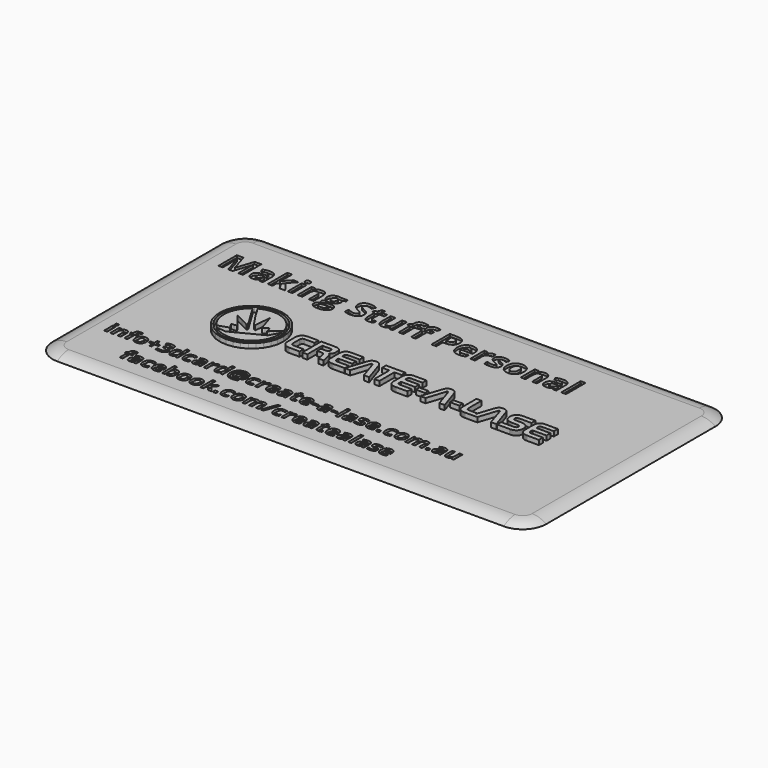
from build123d import *

# Parameters (mm, degrees)
F1_DEPTH     = 1
F0_W         = 1.9434
F0_H         = 0.9282
F4_DEPTH     = 1
F3_TEXT_SIZE = 4.3575753724
F5_DEPTH     = 0.5
F6_TEXT_SIZE = 6.8351726593
F7_DEPTH     = 0.5
F8_T1_DEPTH  = 45
F8_T3_DEPTH  = 95
F8_T6_ANGLE  = 90
F8_T8_ANGLE  = 90
F8_T10_ANGLE = 90
F8_T12_ANGLE = 90


# Not quite as in the source:
# - a fillet or chamfer that OpenCascade refuses, or shapes differently, is made with other operations: its cross-section is extruded or revolved along the edge and cut away or added
# - Text() gives the source's letters only with a copy of the font that has no kerning and outlines rounded to 1/6400 em; it was checked with that copy


with BuildPart() as f1:
    # F0 (on Top) → F1 (new body)
    with BuildSketch(Plane.XY):
        Polygon((-26.8391, 6.60025), (-28.2079, 6.73715), (-29.5767, 6.60025), (-30.8517, 6.20765), (-32.0054, 5.58655), (-33.0107, 4.76385), (-33.8401, 3.76675), (-34.4663, 2.62235), (-34.8621, 1.35775), (-35.0001, 5e-05), (-34.8621, -1.35765), (-34.4663, -2.62235), (-33.8401, -3.76675), (-33.0107, -4.76385), (-32.0054, -5.58655), (-30.8517, -6.20765), (-29.5767, -6.60025), (-28.2079, -6.73715), (-26.8391, -6.60025), (-25.5641, -6.20765), (-24.4103, -5.58655), (-23.4051, -4.76385), (-22.5757, -3.76675), (-21.9494, -2.62235), (-21.5536, -1.35765), (-21.4156, 5e-05), (-21.5536, 1.35775), (-21.9494, 2.62235), (-22.5757, 3.76675), (-23.4051, 4.76385), (-24.4103, 5.58655), (-25.5641, 6.20765), align=None)
        Polygon((-26.9199, -6.21065), (-28.2079, -6.33945), (-29.496, -6.21065), (-30.6957, -5.84125), (-31.7813, -5.25675), (-32.7272, -4.48265), (-33.5077, -3.54445), (-34.0969, -2.46755), (-34.4694, -1.27755), (-34.5992, 5e-05), (-34.4694, 1.27695), (-34.0969, 2.46635), (-33.5077, 3.54275), (-32.7272, 4.48075), (-31.7813, 5.25465), (-30.6957, 5.83905), (-29.496, 6.20845), (-28.2079, 6.33725), (-26.9199, 6.20845), (-25.7205, 5.83905), (-24.6352, 5.25465), (-23.6897, 4.48075), (-22.9096, 3.54275), (-22.3207, 2.46635), (-21.9486, 1.27695), (-21.8188, 5e-05), (-21.9486, -1.27755), (-22.3207, -2.46755), (-22.9096, -3.54445), (-23.6897, -4.48265), (-24.6352, -5.25675), (-25.7205, -5.84125), align=None, mode=Mode.SUBTRACT)
    extrude(amount=F1_DEPTH)



with BuildPart() as f1b:
    # F0 (on Top) → F1, piece 2 (new body)
    with BuildSketch(Plane.XY):
        Polygon((-15.8894, 2.46555), (-18.1095, 2.46555), (-18.2886, 2.45905), (-18.4578, 2.43955), (-18.617, 2.40695), (-18.7664, 2.36145), (-18.9057, 2.30295), (-19.0351, 2.23145), (-19.1544, 2.14705), (-19.2637, 2.04975), (-19.3618, 1.94045), (-19.4468, 1.82115), (-19.5187, 1.69165), (-19.5775, 1.55215), (-19.6231, 1.40255), (-19.6557, 1.24285), (-19.6753, 1.07305), (-19.6818, 0.89315), (-19.6818, -0.98735), (-19.6753, -1.16725), (-19.6557, -1.33725), (-19.6231, -1.49725), (-19.5775, -1.64725), (-19.5187, -1.78725), (-19.4468, -1.91735), (-19.3618, -2.03745), (-19.2637, -2.14755), (-19.1544, -2.24575), (-19.0351, -2.33085), (-18.9057, -2.40295), (-18.7664, -2.46195), (-18.617, -2.50785), (-18.4578, -2.54065), (-18.2886, -2.56035), (-18.1095, -2.56695), (-15.8894, -2.56695), (-15.8894, -1.50825), (-18.0068, -1.50825), (-18.1464, -1.49875), (-18.2678, -1.47015), (-18.3712, -1.42255), (-18.4564, -1.35595), (-18.523, -1.27075), (-18.5706, -1.16745), (-18.5991, -1.04595), (-18.6086, -0.90635), (-18.6086, 0.80495), (-18.5991, 0.94635), (-18.5706, 1.06945), (-18.523, 1.17425), (-18.4564, 1.26055), (-18.3712, 1.32795), (-18.2678, 1.37585), (-18.1464, 1.40455), (-18.0068, 1.41405), (-15.8894, 1.41405), align=None)
    extrude(amount=F1_DEPTH)


with BuildPart() as f1c:
    # F0 (on Top) → F1, piece 3 (new body)
    with BuildSketch(Plane.XY):
        Polygon((-12.5597, 2.46555), (-15.337, 2.46555), (-15.337, -2.56695), (-14.2638, -2.56695), (-14.2638, 1.41405), (-12.6057, 1.41405), (-12.4903, 1.40815), (-12.389, 1.39055), (-12.3018, 1.36105), (-12.2286, 1.31985), (-12.1706, 1.26775), (-12.1291, 1.20575), (-12.1041, 1.13405), (-12.0957, 1.05275), (-12.0957, 0.78195), (-12.1041, 0.70065), (-12.1291, 0.62895), (-12.1706, 0.56695), (-12.2286, 0.51485), (-12.3018, 0.47365), (-12.389, 0.44415), (-12.4903, 0.42655), (-12.6057, 0.42065), (-13.7562, 0.42065), (-13.7562, -0.58735), (-12.6758, -0.58735), (-12.5851, -0.59775), (-12.4999, -0.62925), (-12.4201, -0.68165), (-12.3458, -0.75535), (-12.2796, -0.84665), (-12.226, -0.95185), (-12.1849, -1.07085), (-12.1561, -1.20365), (-11.9083, -2.56695), (-10.7759, -2.56695), (-11.1397, -0.87015), (-11.3379, -0.38065), (-11.4113, -0.28985), (-11.4936, -0.21315), (-11.5848, -0.15065), (-11.6847, -0.10265), (-11.5272, -0.04125), (-11.3917, 0.03965), (-11.2779, 0.13995), (-11.1856, 0.25985), (-11.1142, 0.40125), (-11.0633, 0.56445), (-11.0327, 0.74935), (-11.0225, 0.95605), (-11.0225, 1.35725), (-11.0284, 1.49445), (-11.046, 1.62225), (-11.0754, 1.74075), (-11.1166, 1.84995), (-11.1694, 1.94995), (-11.234, 2.04065), (-11.3103, 2.12235), (-11.3983, 2.19485), (-11.4985, 2.25815), (-11.6116, 2.31305), (-11.7374, 2.35965), (-11.8761, 2.39775), (-12.1921, 2.44855), align=None)
    extrude(amount=F1_DEPTH)


with BuildPart() as f1d:
    # F0 (on Top) → F1, piece 4 (new body)
    with BuildSketch(Plane.XY):
        Polygon((-6.3018, 2.46555), (-8.7902, 2.46555), (-8.9959, 2.45995), (-9.1861, 2.44315), (-9.3609, 2.41505), (-9.5202, 2.37575), (-9.6641, 2.32535), (-9.7926, 2.26355), (-9.9058, 2.19065), (-10.0036, 2.10655), (-10.0877, 2.00875), (-10.1606, 1.89555), (-10.2223, 1.76705), (-10.2728, 1.62315), (-10.312, 1.46385), (-10.3401, 1.28905), (-10.3569, 1.09885), (-10.3625, 0.89315), (-10.3625, -0.98735), (-10.3568, -1.19315), (-10.3399, -1.38345), (-10.3116, -1.55855), (-10.272, -1.71825), (-10.2212, -1.86265), (-10.1591, -1.99175), (-10.0858, -2.10565), (-10.0012, -2.20435), (-9.9034, -2.28935), (-9.7902, -2.36295), (-9.6618, -2.42525), (-9.5181, -2.47625), (-9.359, -2.51595), (-9.1847, -2.54425), (-8.9951, -2.56125), (-8.7902, -2.56695), (-6.3018, -2.56695), (-6.3018, -1.50825), (-8.7092, -1.50825), (-8.8622, -1.50055), (-8.9892, -1.47725), (-9.0901, -1.43835), (-9.1649, -1.38375), (-9.2195, -1.30895), (-9.2583, -1.20795), (-9.2816, -1.08055), (-9.2893, -0.92695), (-9.2893, -0.55105), (-6.3018, -0.55105), (-6.3018, 0.50765), (-9.2893, 0.50765), (-9.2893, 0.82675), (-9.2814, 0.98145), (-9.2577, 1.11005), (-9.2184, 1.21245), (-9.1636, 1.28835), (-9.0882, 1.34315), (-8.9872, 1.38245), (-8.8608, 1.40615), (-8.7092, 1.41405), (-6.3018, 1.41405), align=None)
    extrude(amount=F1_DEPTH)


with BuildPart() as f1e:
    # F0 (on Top) → F1, piece 5 (new body)
    with BuildSketch(Plane.XY):
        Polygon((-1.0953, -2.56695), (-2.4875, 1.63885), (-2.565, 1.85635), (-2.6632, 2.04495), (-2.7821, 2.20445), (-2.9214, 2.33495), (-3.0816, 2.43645), (-3.2633, 2.50905), (-3.4664, 2.55255), (-3.6913, 2.56705), (-3.9154, 2.55325), (-4.1162, 2.51175), (-4.2938, 2.44265), (-4.4478, 2.34585), (-4.5826, 2.21875), (-4.7024, 2.05855), (-4.8069, 1.86525), (-4.8962, 1.63885), (-6.28, -2.56695), (-5.1403, -2.56695), (-3.8786, 1.33435), (-3.8061, 1.46725), (-3.6913, 1.50835), (-3.5692, 1.46605), (-3.493, 1.33185), (-2.2325, -2.56695), align=None)
    extrude(amount=F1_DEPTH)


with BuildPart() as f1f:
    # F0 (on Top) → F1, piece 6 (new body)
    with BuildSketch(Plane.XY):
        Polygon((2.5922, 2.46555), (-1.5339, 2.46555), (-1.5339, 1.41405), (-0.0038, 1.41405), (-0.0038, -2.56695), (1.0694, -2.56695), (1.0694, 1.41405), (2.5922, 1.41405), align=None)
    extrude(amount=F1_DEPTH)


with BuildPart() as f1g:
    # F0 (on Top) → F1, piece 7 (new body)
    with BuildSketch(Plane.XY):
        Polygon((7.0602, 2.46555), (4.5718, 2.46555), (4.3661, 2.45995), (4.1759, 2.44315), (4.0011, 2.41505), (3.8418, 2.37575), (3.6979, 2.32535), (3.5694, 2.26355), (3.4562, 2.19065), (3.3584, 2.10655), (3.2743, 2.00875), (3.2014, 1.89555), (3.1397, 1.76705), (3.0892, 1.62315), (3.05, 1.46385), (3.0219, 1.28905), (3.0051, 1.09885), (2.9995, 0.89315), (2.9995, -0.98735), (3.0052, -1.19315), (3.0221, -1.38345), (3.0504, -1.55855), (3.09, -1.71825), (3.1408, -1.86265), (3.2029, -1.99175), (3.2762, -2.10565), (3.3608, -2.20435), (3.4586, -2.28935), (3.5718, -2.36295), (3.7002, -2.42525), (3.8439, -2.47625), (4.003, -2.51595), (4.1773, -2.54425), (4.3669, -2.56125), (4.5718, -2.56695), (7.0602, -2.56695), (7.0602, -1.50825), (4.6528, -1.50825), (4.4998, -1.50055), (4.3728, -1.47725), (4.2719, -1.43835), (4.1971, -1.38375), (4.1425, -1.30895), (4.1037, -1.20795), (4.0804, -1.08055), (4.0727, -0.92695), (4.0727, -0.55105), (7.0602, -0.55105), (7.0602, 0.50765), (4.0727, 0.50765), (4.0727, 0.82675), (4.0806, 0.98145), (4.1043, 1.11005), (4.1436, 1.21245), (4.1984, 1.28835), (4.2738, 1.34315), (4.3748, 1.38245), (4.5012, 1.40615), (4.6528, 1.41405), (7.0602, 1.41405), align=None)
    extrude(amount=F1_DEPTH)


with BuildPart() as f1h:
    # F0 (on Top) → F1, piece 8 (new body)
    with BuildSketch(Plane.XY):
        with Locations((8.7063, -0.74685)):
            Rectangle(F0_W, F0_H)
    extrude(amount=F1_DEPTH)


with BuildPart() as f1i:
    # F0 (on Top) → F1, piece 9 (new body)
    with BuildSketch(Plane.XY):
        Polygon((14.9509, -2.56695), (13.5587, 1.63885), (13.4812, 1.85635), (13.383, 2.04495), (13.2641, 2.20445), (13.1248, 2.33495), (12.9646, 2.43645), (12.7829, 2.50905), (12.5798, 2.55255), (12.3549, 2.56705), (12.1308, 2.55325), (11.93, 2.51175), (11.7524, 2.44265), (11.5984, 2.34585), (11.4636, 2.21875), (11.3438, 2.05855), (11.2393, 1.86525), (11.15, 1.63885), (9.7662, -2.56695), (10.9059, -2.56695), (12.1676, 1.33435), (12.2401, 1.46725), (12.3549, 1.50835), (12.477, 1.46605), (12.5532, 1.33185), (13.8137, -2.56695), align=None)
    extrude(amount=F1_DEPTH)


with BuildPart() as f1j:
    # F0 (on Top) → F1, piece 10 (new body)
    with BuildSketch(Plane.XY):
        with Locations((16.0109, -0.74685)):
            Rectangle(F0_W, F0_H)
    extrude(amount=F1_DEPTH)


with BuildPart() as f1k:
    # F0 (on Top) → F1, piece 11 (new body)
    with BuildSketch(Plane.XY):
        Polygon((18.7604, 2.46555), (17.6872, 2.46555), (17.6872, -0.98735), (17.6929, -1.19315), (17.7101, -1.38345), (17.7386, -1.55855), (17.7786, -1.71825), (17.8299, -1.86265), (17.8927, -1.99175), (17.9667, -2.10565), (18.0522, -2.20435), (18.1509, -2.28935), (18.265, -2.36295), (18.3943, -2.42525), (18.5389, -2.47625), (18.6989, -2.51595), (18.8741, -2.54425), (19.0646, -2.56125), (19.2704, -2.56695), (20.7606, -2.56695), (20.9793, -1.902252457), (20.9793, -1.50825), (19.3477, -1.50825), (19.1946, -1.50035), (19.0668, -1.47665), (18.9643, -1.43735), (18.8873, -1.38255), (18.8318, -1.30715), (18.7921, -1.20595), (18.7683, -1.07915), (18.7604, -0.92695), align=None)
        Polygon((22.1444, 1.63885), (20.9793, -1.902252457), (20.9793, -2.56695), (21.9003, -2.56695), (23.162, 1.33435), (23.2345, 1.46725), (23.3493, 1.50835), (23.4714, 1.46605), (23.5476, 1.33185), (24.8082, -2.56695), (25.9454, -2.56695), (24.5531, 1.63885), (24.4756, 1.85635), (24.3774, 2.04495), (24.2585, 2.20445), (24.1192, 2.33495), (23.959, 2.43645), (23.7773, 2.50905), (23.5742, 2.55255), (23.3493, 2.56705), (23.1252, 2.55325), (22.9244, 2.51175), (22.7468, 2.44265), (22.5928, 2.34585), (22.458, 2.21875), (22.3382, 2.05855), (22.2337, 1.86525), align=None)
        Polygon((20.9793, -2.56695), (20.9793, -1.902252457), (20.7606, -2.56695), align=None)
    extrude(amount=F1_DEPTH)


with BuildPart() as f1l:
    # F0 (on Top) → F1, piece 12 (new body)
    with BuildSketch(Plane.XY):
        Polygon((30.2432, 2.46555), (27.6327, 2.46555), (27.4486, 2.45925), (27.2745, 2.44035), (27.1102, 2.40885), (26.9559, 2.36475), (26.8115, 2.30805), (26.6772, 2.23865), (26.5529, 2.15655), (26.4386, 2.06185), (26.3362, 1.95615), (26.2474, 1.84135), (26.1722, 1.71725), (26.1107, 1.58385), (26.0627, 1.44125), (26.0285, 1.28925), (26.008, 1.12795), (26.0011, 0.95725), (26.008, 0.78735), (26.0285, 0.62665), (26.0627, 0.47505), (26.1107, 0.33255), (26.1722, 0.19925), (26.2474, 0.07505), (26.3362, -0.04015), (26.4386, -0.14615), (26.5529, -0.24095), (26.6772, -0.32315), (26.8115, -0.39275), (26.9559, -0.44975), (27.1102, -0.49405), (27.2745, -0.52565), (27.4486, -0.54475), (27.6327, -0.55105), (28.7651, -0.55105), (28.9097, -0.55855), (29.0354, -0.58085), (29.1423, -0.61785), (29.2304, -0.66955), (29.2993, -0.73685), (29.3484, -0.81925), (29.3777, -0.91675), (29.3875, -1.02965), (29.3777, -1.14115), (29.3484, -1.23795), (29.2993, -1.32005), (29.2304, -1.38735), (29.1423, -1.44045), (29.0354, -1.47815), (28.9097, -1.50075), (28.7651, -1.50825), (26.1027, -1.50825), (26.1027, -2.56695), (28.7398, -2.56695), (28.9381, -2.56065), (29.125, -2.54155), (29.3007, -2.50975), (29.4652, -2.46525), (29.6184, -2.40805), (29.7605, -2.33795), (29.8914, -2.25525), (30.0112, -2.15965), (30.1183, -2.05285), (30.211, -1.93615), (30.2895, -1.80975), (30.3538, -1.67355), (30.4038, -1.52745), (30.4394, -1.37145), (30.4609, -1.20545), (30.468, -1.02965), (30.4609, -0.85385), (30.4394, -0.68785), (30.4038, -0.53185), (30.3538, -0.38575), (30.2895, -0.24955), (30.211, -0.12315), (30.1183, -0.00645), (30.0112, 0.10035), (29.8914, 0.19595), (29.7605, 0.27865), (29.6184, 0.34875), (29.4652, 0.40595), (29.3007, 0.45045), (29.125, 0.48225), (28.9381, 0.50135), (28.7398, 0.50765), (27.6122, 0.50765), (27.4878, 0.51465), (27.3794, 0.53595), (27.287, 0.57135), (27.2109, 0.62125), (27.1513, 0.68445), (27.1086, 0.76155), (27.0829, 0.85255), (27.0743, 0.95725), (27.0829, 1.06355), (27.1086, 1.15595), (27.1513, 1.23445), (27.2109, 1.29925), (27.287, 1.34925), (27.3794, 1.38515), (27.4878, 1.40685), (27.6122, 1.41405), (30.2432, 1.41405), align=None)
    extrude(amount=F1_DEPTH)


with BuildPart() as f1m:
    # F0 (on Top) → F1, piece 13 (new body)
    with BuildSketch(Plane.XY):
        Polygon((35.0001, 2.46555), (32.5117, 2.46555), (32.306, 2.45995), (32.1158, 2.44315), (31.941, 2.41505), (31.7817, 2.37575), (31.6378, 2.32535), (31.5093, 2.26355), (31.3961, 2.19065), (31.2983, 2.10655), (31.2142, 2.00875), (31.1413, 1.89555), (31.0796, 1.76705), (31.0291, 1.62315), (30.9899, 1.46385), (30.9618, 1.28905), (30.945, 1.09885), (30.9394, 0.89315), (30.9394, -0.98735), (30.9451, -1.19315), (30.962, -1.38345), (30.9903, -1.55855), (31.0299, -1.71825), (31.0807, -1.86265), (31.1428, -1.99175), (31.2161, -2.10565), (31.3007, -2.20435), (31.3985, -2.28935), (31.5117, -2.36295), (31.6401, -2.42525), (31.7838, -2.47625), (31.9429, -2.51595), (32.1172, -2.54425), (32.3068, -2.56125), (32.5117, -2.56695), (35.0001, -2.56695), (35.0001, -1.50825), (32.5927, -1.50825), (32.4397, -1.50055), (32.3127, -1.47725), (32.2118, -1.43835), (32.137, -1.38375), (32.0824, -1.30895), (32.0436, -1.20795), (32.0203, -1.08055), (32.0126, -0.92695), (32.0126, -0.55105), (35.0001, -0.55105), (35.0001, 0.50765), (32.0126, 0.50765), (32.0126, 0.82675), (32.0205, 0.98145), (32.0442, 1.11005), (32.0835, 1.21245), (32.1383, 1.28835), (32.2137, 1.34315), (32.3147, 1.38245), (32.4411, 1.40615), (32.5927, 1.41405), (35.0001, 1.41405), align=None)
    extrude(amount=F1_DEPTH)


with BuildPart() as f1n:
    # F0 (on Top) → F1, piece 14 (new body)
    with BuildSketch(Plane.XY):
        Polygon((-23.8806, 0.40645), (-22.5791, 1.59085), (-22.912, 2.47015), (-23.3776, 3.27525), (-23.9625, 3.99285), (-24.6535, 4.60985), (-25.437, 5.11275), (-26.2999, 5.48835), (-27.2287, 5.72355), (-28.2101, 5.80485), (-28.582, 5.79335), (-28.9478, 5.75925), (-29.3067, 5.70325), (-29.6581, 5.62605), (-30.0012, 5.52825), (-30.3352, 5.41055), (-30.6594, 5.27365), (-30.973, 5.11805), (-29.459, 2.60145), (-27.98, 0.39115), (-27.5856, 0.22165), (-27.2636, 3.80545), (-26.0913, 0.10215), (-25.6378, 0.40645), (-24.9498, 0.87145), (-24.6409, -0.26295), (-24.3473, -0.00215), align=None)
    extrude(amount=F1_DEPTH)


with BuildPart() as f1o:
    # F0 (on Top) → F1, piece 15 (new body)
    with BuildSketch(Plane.XY):
        Polygon((-28.8302, -0.32165), (-28.7557, -0.16085), (-30.2259, 2.24935), (-31.6785, 4.67475), (-32.1961, 4.24985), (-32.6611, 3.76915), (-33.0683, 3.23775), (-33.4127, 2.66065), (-33.6894, 2.04305), (-33.8933, 1.38995), (-34.0193, 0.70655), (-34.0624, -0.00215), (-34.0368, -0.54765), (-33.9615, -1.07925), (-33.8387, -1.59455), (-33.6707, -2.09115), (-33.4598, -2.56685), (-33.2083, -3.01915), (-32.9183, -3.44585), (-32.5922, -3.84445), (-31.9962, -3.64895), (-30.3244, -3.09685), (-30.6553, -2.50795), (-30.984, -1.91685), (-30.3924, -1.85375), (-29.7986, -1.78645), (-30.962, -0.29775), (-32.1277, 1.19095), (-30.5151, 0.35645), (-28.9046, -0.48025), align=None)
    extrude(amount=F1_DEPTH)


with BuildPart() as f1p:
    # F0 (on Top) → F1, piece 16 (new body)
    with BuildSketch(Plane.XY):
        Polygon((-22.4746, -1.17135), (-22.3556, -0.00215), (-22.4301, 0.92585), (-22.5331, 0.74105), (-23.6089, -1.32135), (-30.0308, -4.64215), (-31.8494, -4.42255), (-32.0291, -4.39865), (-31.6305, -4.71125), (-31.205, -4.98915), (-30.7549, -5.23005), (-30.2823, -5.43205), (-29.7893, -5.59285), (-29.2782, -5.71035), (-28.7511, -5.78245), (-28.2101, -5.80695), (-27.0307, -5.68895), (-25.9319, -5.35045), (-24.9375, -4.81495), (-24.0709, -4.10585), (-23.3559, -3.24655), (-22.8159, -2.26055), align=None)
    extrude(amount=F1_DEPTH)


with BuildPart() as f1_1:
    add(f1.part)

    add(f1b.part)  # F4 merges F1b

    add(f1c.part)  # F4 merges F1c

    add(f1d.part)  # F4 merges F1d

    add(f1e.part)  # F4 merges F1e

    add(f1f.part)  # F4 merges F1f

    add(f1g.part)  # F4 merges F1g

    add(f1h.part)  # F4 merges F1h

    add(f1i.part)  # F4 merges F1i

    add(f1j.part)  # F4 merges F1j

    add(f1k.part)  # F4 merges F1k

    add(f1l.part)  # F4 merges F1l

    add(f1m.part)  # F4 merges F1m

    add(f1n.part)  # F4 merges F1n

    add(f1o.part)  # F4 merges F1o

    add(f1p.part)  # F4 merges F1p
    # F2 (on Top) → F4 (join)
    with BuildSketch(Plane.XY):
        with BuildLine():
            Line((-47.5, -27.5), (47.5, -27.5))
            ThreePointArc((47.5, -27.5), (51.0355339059, -26.0355339059), (52.5, -22.5))
            Line((52.5, -22.5), (52.5, 22.5))
            ThreePointArc((52.5, 22.5), (51.0355339059, 26.0355339059), (47.5, 27.5))
            Line((47.5, 27.5), (-47.5, 27.5))
            ThreePointArc((-47.5, 27.5), (-51.0355339059, 26.0355339059), (-52.5, 22.5))
            Line((-52.5, 22.5), (-52.5, -22.5))
            ThreePointArc((-52.5, -22.5), (-51.0355339059, -26.0355339059), (-47.5, -27.5))
        make_face()
    extrude(amount=-F4_DEPTH)

    # F3 (on face) → F5 (cut)
    with BuildSketch(Plane.XY):
        with Locations((-47.5, -15.5)):
            Text('info+3dcard@create-a-lase.com.au', F3_TEXT_SIZE, font='Open Sans', font_style=FontStyle.BOLD, text_align=(TextAlign.LEFT, TextAlign.BOTTOM))
        with Locations((-39.5739789202, -21.4263025065)):
            Text('facebook.com/createalase', F3_TEXT_SIZE, font='Open Sans', font_style=FontStyle.BOLD, text_align=(TextAlign.LEFT, TextAlign.BOTTOM))
    extrude(amount=-F5_DEPTH, mode=Mode.SUBTRACT)

    # F6 (on face) → F7 (cut)
    with BuildSketch(Plane.XY):
        with Locations((-47.5, 14.5786756853)):
            Text('Making Stuff Personal', F6_TEXT_SIZE, font='Open Sans', font_style=FontStyle.BOLD, text_align=(TextAlign.LEFT, TextAlign.BOTTOM))
    extrude(amount=-F7_DEPTH, mode=Mode.SUBTRACT)

    # F8: fillet of radius 5 on 1 edges, made by hand

    # F8_s2 → F8_t1 (cut)
    with BuildSketch(Plane.XZ.offset(-22.5)):
        with BuildLine():
            ThreePointArc((-49.5, 0), (-51.0811388301, -0.2565835097), (-52.5, -1))
            Line((-52.5, -1), (-52.5, 0))
            Line((-52.5, 0), (-49.5, 0))
        make_face()
        with BuildLine():
            ThreePointArc((49.5, 0), (51.0811388301, -0.2565835097), (52.5, -1))
            Line((52.5, -1), (52.5, 0))
            Line((52.5, 0), (49.5, 0))
        make_face()
    extrude(amount=F8_T1_DEPTH, mode=Mode.SUBTRACT)

    # F8_s4 → F8_t3 (cut)
    with BuildSketch(Plane.YZ.offset(-47.5)):
        with BuildLine():
            ThreePointArc((-27.5, -1), (-26.0811388301, -0.2565835097), (-24.5, 0))
            Line((-24.5, 0), (-27.5, 0))
            Line((-27.5, 0), (-27.5, -1))
        make_face()
        with BuildLine():
            ThreePointArc((24.5, 0), (26.0811388301, -0.2565835097), (27.5, -1))
            Line((27.5, -1), (27.5, 0))
            Line((27.5, 0), (24.5, 0))
        make_face()
    extrude(amount=F8_T3_DEPTH, mode=Mode.SUBTRACT)

    # F8_s5 → F8_t6 (revolve, cut)
    with BuildSketch(Plane.YZ.offset(-47.5)):
        with BuildLine():
            ThreePointArc((24.5, 0), (26.0811388301, -0.2565835097), (27.5, -1))
            Line((27.5, -1), (27.5, 0))
            Line((27.5, 0), (24.5, 0))
        make_face()
    revolve(axis=Axis((-47.5, 22.5, 0), (0, 0, 1)), revolution_arc=F8_T6_ANGLE, mode=Mode.SUBTRACT)

    # F8_s7 → F8_t8 (revolve, cut)
    with BuildSketch(Plane.XZ.offset(22.5)):
        with BuildLine():
            ThreePointArc((-52.5, -1), (-51.0811388301, -0.2565835097), (-49.5, 0))
            Line((-49.5, 0), (-52.5, 0))
            Line((-52.5, 0), (-52.5, -1))
        make_face()
    revolve(axis=Axis((-47.5, -22.5, 0), (0, 0, 1)), revolution_arc=F8_T8_ANGLE, mode=Mode.SUBTRACT)

    # F8_s9 → F8_t10 (revolve, cut)
    with BuildSketch(Plane.YZ.offset(47.5)):
        with BuildLine():
            ThreePointArc((-27.5, -1), (-26.0811388301, -0.2565835097), (-24.5, 0))
            Line((-24.5, 0), (-27.5, 0))
            Line((-27.5, 0), (-27.5, -1))
        make_face()
    revolve(axis=Axis((47.5, -22.5, 0), (0, 0, 1)), revolution_arc=F8_T10_ANGLE, mode=Mode.SUBTRACT)

    # F8_s11 → F8_t12 (revolve, cut)
    with BuildSketch(Plane.XZ.offset(-22.5)):
        with BuildLine():
            ThreePointArc((49.5, 0), (51.0811388301, -0.2565835097), (52.5, -1))
            Line((52.5, -1), (52.5, 0))
            Line((52.5, 0), (49.5, 0))
        make_face()
    revolve(axis=Axis((47.5, 22.5, 0), (0, 0, 1)), revolution_arc=F8_T12_ANGLE, mode=Mode.SUBTRACT)


solid = f1_1.part
